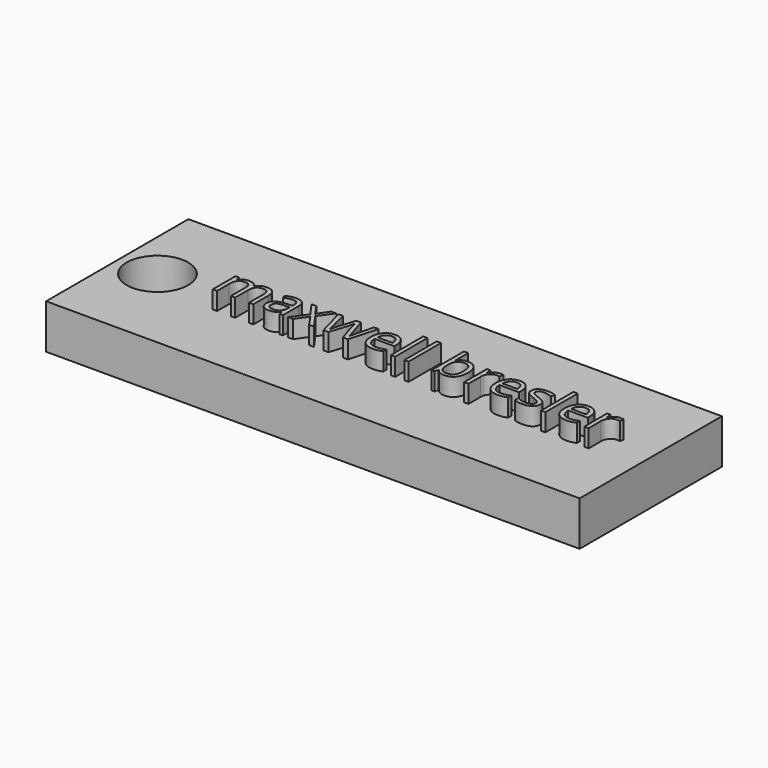
from build123d import *

# Parameters (mm, degrees)
F0_W         = 76.2
F0_H         = 25.4
F1_DEPTH     = 6.35
F3_TEXT_SIZE = 7.5948748013
F4_DEPTH     = 2.54
F2_R         = 4.3931640916
F5_DEPTH     = 127


# Not quite as in the source:
# - Text() gives the source's letters only with a copy of the font that has no kerning and outlines rounded to 1/6400 em; it was checked with that copy


with BuildPart() as f1:
    # F0 (on Top) → F1 (new body)
    with BuildSketch(Plane.XY):
        with Locations((9.2319250107, 2.6430218974)):
            Rectangle(F0_W, F0_H)
    extrude(amount=F1_DEPTH)

    # F3 (on face) → F4 (join)
    with BuildSketch(Plane.XY.offset(6.35)):
        with Locations((-13.764071261, 0)):
            Text('maxwell bresler', F3_TEXT_SIZE, font='Open Sans', text_align=(TextAlign.LEFT, TextAlign.BOTTOM))
    extrude(amount=F4_DEPTH)

    # F2 (on face) → F5 (cut)
    with BuildSketch(Plane.XY.offset(6.35)):
        with Locations((-23.312266916, 2.8780577704)):
            Circle(F2_R)
    extrude(amount=-F5_DEPTH, mode=Mode.SUBTRACT)


solid = f1.part
